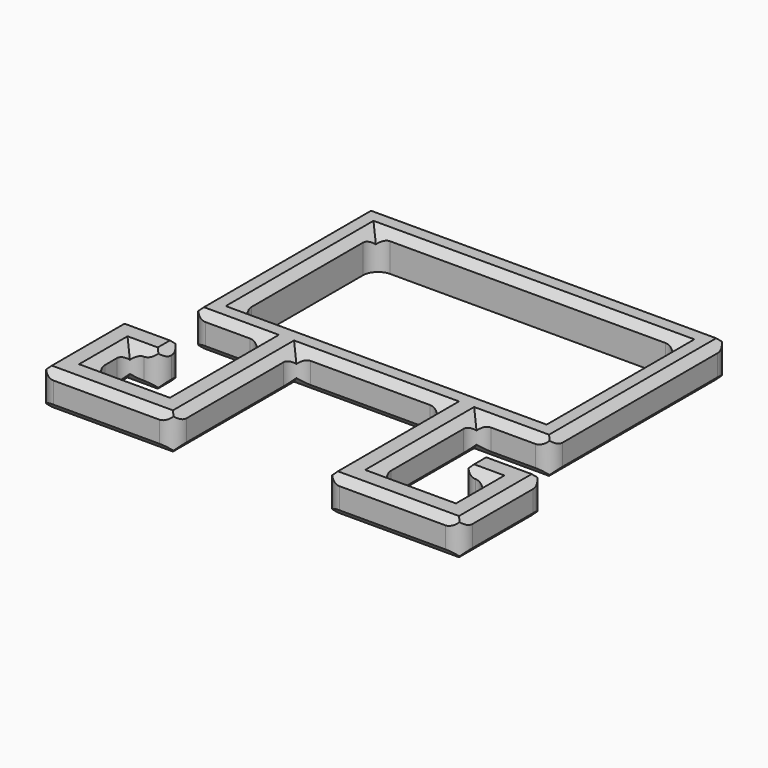
from build123d import *

# Parameters (mm, degrees)
F0_W     = 101
F0_H     = 56
F1_DEPTH = 12
F2_SIZE  = 2.5
F3_R     = 4.99999


# Not quite as in the source:
# - a fillet or chamfer is up to 0.001 mm smaller than in the source, because OpenCascade refuses the exact size


with BuildPart() as f1:
    # F0 (on Top) → F1 (new body)
    with BuildSketch(Plane.XY):
        Polygon((75.1021924019, 82.3358418196), (-43.8978075981, 82.3358418196), (-43.8978075981, 8.3358418196), (-19.1478075981, 8.3358418196), (-9.1478075981, 8.3358418196), (15.6021924019, 8.3358418196), (40.3521924019, 8.3358418196), (50.3521924019, 8.3358418196), (75.1021924019, 8.3358418196), align=None)
        with Locations((15.6021924019, 45.3358418196)):
            Rectangle(F0_W, F0_H, mode=Mode.SUBTRACT)
        Polygon((-9.1478075981, 8.3358418196), (-19.1478075981, 8.3358418196), (-19.1478075981, -31.6641581804), (-44.1478075981, -31.6641581804), (-44.1478075981, -16.6641581804), (-34.1478075981, -16.6641581804), (-34.1478075981, -6.6641581804), (-44.1478075981, -6.6641581804), (-54.1478075981, -6.6641581804), (-54.1478075981, -41.6641581804), (-9.1478075981, -41.6641581804), align=None)
        Polygon((50.3521924019, -31.6641581804), (50.3521924019, 8.3358418196), (40.3521924019, 8.3358418196), (40.3521924019, -41.6641581804), (85.3521924019, -41.6641581804), (85.3521924019, -6.6641581804), (75.3521924019, -6.6641581804), (65.3521924019, -6.6641581804), (65.3521924019, -16.6641581804), (75.3521924019, -16.6641581804), (75.3521924019, -31.6641581804), align=None)
    extrude(amount=F1_DEPTH)

    # F2
    f2_edges = [f1.edges().sort_by_distance(p)[0] for p in [
        (-43.897808, 45.335842, 0),
        (15.602192, 82.335842, 0),
        (75.102192, 45.335842, 0),
        (62.727192, 8.335842, 0),
        (50.352192, -11.664158, 0),
        (62.852192, -31.664158, 0),
        (75.352192, -24.164158, 0),
        (70.352192, -16.664158, 0),
        (65.352192, -11.664158, 0),
        (75.352192, -6.664158, 0),
        (85.352192, -24.164158, 0),
        (62.852192, -41.664158, 0),
        (-31.522808, 8.335842, 0),
        (40.352192, -16.664158, 0),
        (-9.147808, -16.664158, 0),
        (-31.647808, -41.664158, 0),
        (-54.147808, -24.164158, 0),
        (-44.147808, -6.664158, 0),
        (-31.647808, -31.664158, 0),
        (-19.147808, -11.664158, 0),
        (-31.522808, 8.335842, 12),
        (62.727192, 8.335842, 12),
        (15.602192, 82.335842, 12),
        (-43.897808, 45.335842, 12),
        (-19.147808, -11.664158, 12),
        (-31.647808, -31.664158, 12),
        (-44.147808, -24.164158, 12),
        (-39.147808, -16.664158, 12),
        (-34.147808, -11.664158, 12),
        (-44.147808, -6.664158, 12),
        (-54.147808, -24.164158, 12),
        (-31.647808, -41.664158, 12),
        (-9.147808, -16.664158, 12),
        (15.602192, 8.335842, 12),
        (40.352192, -16.664158, 12),
        (62.852192, -41.664158, 12),
        (85.352192, -24.164158, 12),
        (75.352192, -6.664158, 12),
        (65.352192, -11.664158, 12),
        (70.352192, -16.664158, 12),
        (75.352192, -24.164158, 12),
        (62.852192, -31.664158, 12),
        (50.352192, -11.664158, 12),
        (75.102192, 45.335842, 12),
        (15.602192, 17.335842, 12),
        (-34.897808, 45.335842, 12),
        (15.602192, 73.335842, 12),
        (66.102192, 45.335842, 12),
        (-39.147808, -16.664158, 0),
        (-44.147808, -24.164158, 0),
        (-34.147808, -11.664158, 0),
        (15.602192, 8.335842, 0),
    ]]
    chamfer(f2_edges, length=F2_SIZE)

    # F3 (radius 5 in the source; OpenCascade refuses exactly that, so slightly less here)
    f3_edges = [f1.edges().sort_by_distance(p)[0] for p in [
        (-34.897808, 73.335842, 4.75),
        (-34.897808, 17.335842, 4.75),
        (66.102192, 17.335842, 4.75),
        (66.102192, 73.335842, 4.75),
        (75.102192, 8.335842, 6),
        (-43.897808, 8.335842, 6),
        (-43.897808, 82.335842, 6),
        (75.102192, 82.335842, 6),
        (-19.147808, 8.335842, 6),
        (-9.147808, 8.335842, 6),
        (40.352192, 8.335842, 6),
        (50.352192, 8.335842, 6),
        (-9.147808, -41.664158, 6),
        (-54.147808, -41.664158, 6),
        (-54.147808, -6.664158, 6),
        (-34.147808, -6.664158, 6),
        (-34.147808, -16.664158, 6),
        (-44.147808, -16.664158, 6),
        (-44.147808, -31.664158, 6),
        (-19.147808, -31.664158, 6),
        (40.352192, -41.664158, 6),
        (85.352192, -41.664158, 6),
        (85.352192, -6.664158, 6),
        (65.352192, -6.664158, 6),
        (65.352192, -16.664158, 6),
        (75.352192, -16.664158, 6),
        (50.352192, -31.664158, 6),
        (75.352192, -31.664158, 6),
    ]]
    fillet(f3_edges, radius=F3_R)


solid = f1.part
